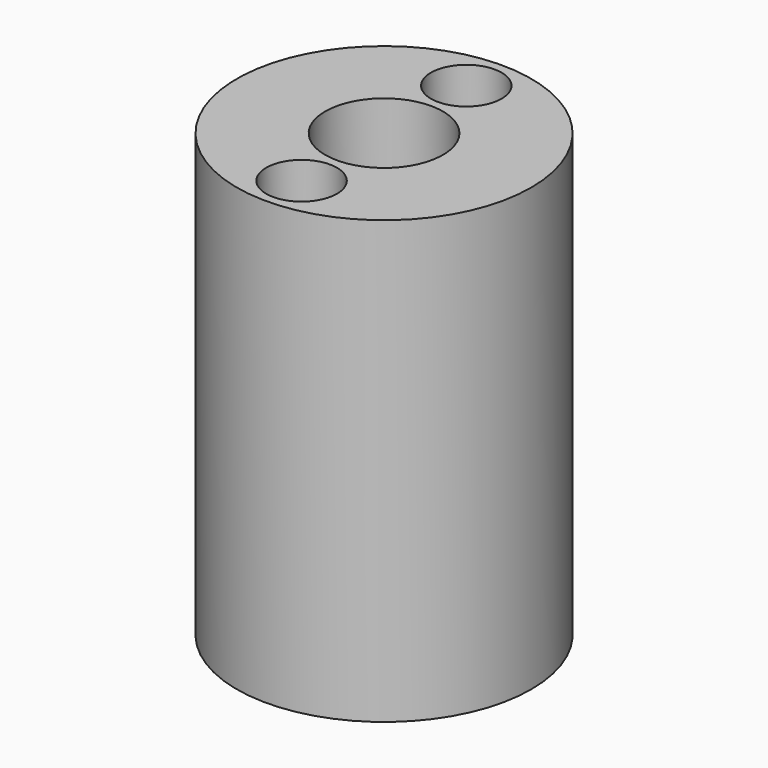
from build123d import *

# Parameters (mm, degrees)
F0_R      = 6.35
F1_DEPTH  = 19.05
F3_D      = 5.08
F8_D      = 3.048
F8_DEPTH  = 2.54
F8_TIP    = 0.9157115834
F9_D      = 3.048
F9_DEPTH  = 2.54
F9_TIP    = 0.9157115834
F11_D     = 11.938
F11_DEPTH = 12.7
F11_TIP   = 3.586537035


# Not quite as in the source:
# - the program builds the solid bodies; features that only make, move or delete a surface that nothing else refers to are left out


with BuildPart() as f1:
    # F0 (on Top) → F1 (new body)
    with BuildSketch(Plane.XY):
        Circle(F0_R)
    extrude(amount=F1_DEPTH)

    # F3 (through all)
    with Locations(Plane(origin=(0, 0, 0), x_dir=(1, 0, 0), z_dir=(0, 0, -1))):
        with Locations((0, 0)):
            Hole(F3_D / 2)

    # F8
    with Locations(Plane.XY.offset(19.05)):
        with Locations((0, 4.4337138534)):
            Hole(F8_D / 2, depth=F8_DEPTH)
            with Locations((0, 0, -(F8_DEPTH + F8_TIP / 2))):  # 118° drill point
                Cone(0, F8_D / 2, F8_TIP, mode=Mode.SUBTRACT)

    # F9
    with Locations(Plane.XY.offset(19.05)):
        with Locations((0, -4.445)):
            Hole(F9_D / 2, depth=F9_DEPTH)
            with Locations((0, 0, -(F9_DEPTH + F9_TIP / 2))):  # 118° drill point
                Cone(0, F9_D / 2, F9_TIP, mode=Mode.SUBTRACT)

    # F11
    with Locations(Plane(origin=(0, 0, 0), x_dir=(1, 0, 0), z_dir=(0, 0, -1))):
        with Locations((0, 0)):
            Hole(F11_D / 2, depth=F11_DEPTH)
            with Locations((0, 0, -(F11_DEPTH + F11_TIP / 2))):  # 118° drill point
                Cone(0, F11_D / 2, F11_TIP, mode=Mode.SUBTRACT)


solid = f1.part
